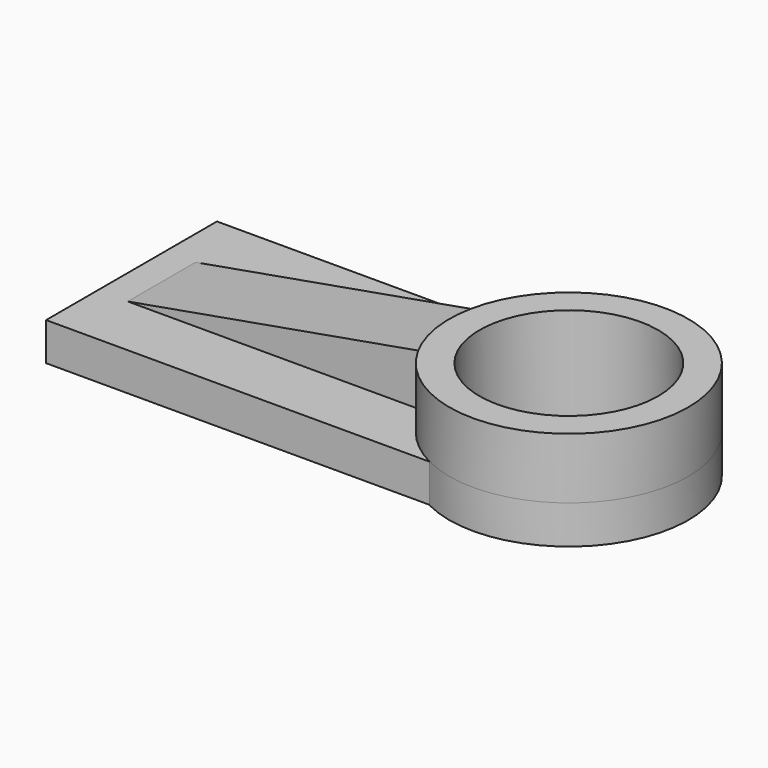
from build123d import *

# Parameters (mm, degrees)
F6_W        = 152.1180570126
F6_H        = 74.284017086
F0_DEPTH    = 13.2086668164
F1_DEPTH    = 13.3642852306
F2_W        = 151.2780189514
F2_H        = 29.4950902462
F8_DEPTH    = 20.6191111356
F3_T4_DEPTH = 689.5239445372
F4_DEPTH    = 34.5556028187
F5_R        = 31.0991112757
F9_DEPTH    = 34.5566028187


# Not quite as in the source:
# - a fillet or chamfer that OpenCascade refuses, or shapes differently, is made with other operations: its cross-section is extruded or revolved along the edge and cut away or added


with BuildPart() as f0:
    # F6 (on Top) → F0 (new body)
    with BuildSketch(Plane.XY):
        Rectangle(F6_W, F6_H)
    extrude(amount=F0_DEPTH)

    # F7 (on face) → F1 (join)
    with BuildSketch(Plane.XY.offset(13.2086668164)):
        with BuildLine():
            Line((76.0590285063, 37.142008543), (57.3713417563, 37.142008543))
            ThreePointArc((57.3713417563, 37.142008543), (34.4806875741, 0), (57.3713417563, -37.142008543))
            Line((57.3713417563, -37.142008543), (76.0590285063, -37.142008543))
            Line((76.0590285063, -37.142008543), (76.0590285063, 37.142008543))
        make_face()
        with BuildLine():
            ThreePointArc((57.3713417563, -37.142008543), (97.873650022, -35.396055187), (117.6373694385, 0))
            ThreePointArc((117.6373694385, 0), (97.873650022, 35.396055187), (57.3713417563, 37.142008543))
            Line((57.3713417563, 37.142008543), (76.0590285063, 37.142008543))
            Line((76.0590285063, 37.142008543), (76.0590285063, -37.142008543))
            Line((76.0590285063, -37.142008543), (57.3713417563, -37.142008543))
        make_face()
    extrude(amount=-F1_DEPTH)

    # F2 (on face) → F8 (join)
    with BuildSketch(Plane.XY.offset(13.2086668164)):
        Rectangle(F2_W, F2_H)
    extrude(amount=F8_DEPTH)

    # F3: chamfer of 127 x 22.39352655 on 1 edges, made by hand


with BuildPart() as f3_tool2:
    # F3_s3 → F3_t4 (new body)
    with BuildSketch(Plane.XZ.offset(-344.7619722686)):
        Polygon((-75.6390094757, 11.434251402), (51.3609905243, 33.827777952), (-75.6390094757, 33.827777952), align=None)
    extrude(amount=F3_T4_DEPTH)

    split(bisect_by=Plane.XY.offset(13.2086668164), keep=Keep.TOP)


with BuildPart() as f0_1:
    add(f0.part)

    # F3_t1: cut F3_tool2
    add(f3_tool2.part, mode=Mode.SUBTRACT)

    # F4 (add): a face of the model
    f4_faces = [f0_1.faces().sort_by_distance(p)[0] for p in [
        (76.0590285063, 0, -0.1556184143),
    ]]
    extrude(f4_faces, amount=-F4_DEPTH)

    # F5 (on face) → F9 (cut, through all)
    with BuildSketch(Plane.XY.offset(34.3999844044)):
        with Locations((76.0590285063, 0)):
            Circle(F5_R)
    extrude(amount=-F9_DEPTH, mode=Mode.SUBTRACT)


solid = f0_1.part
